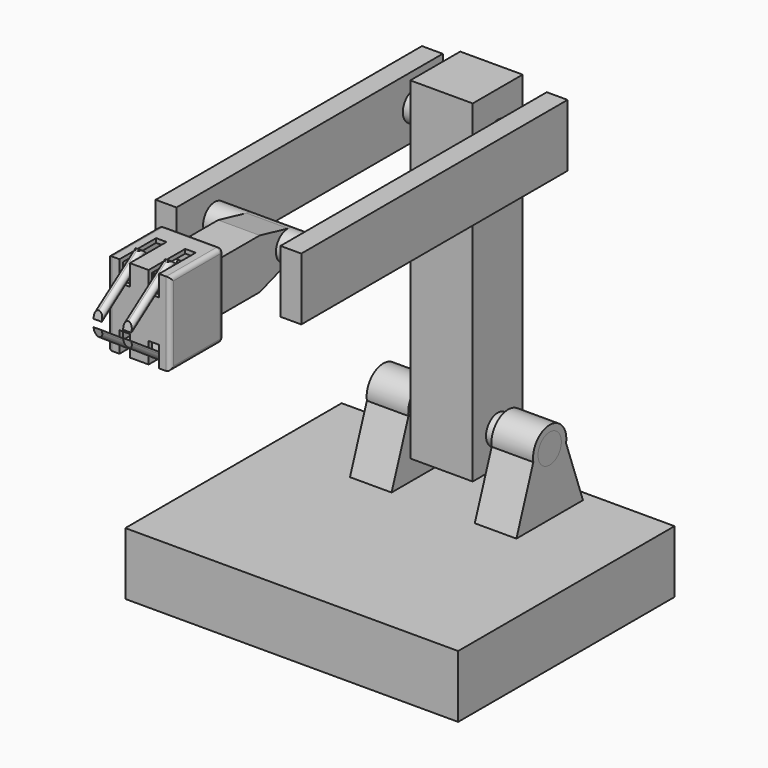
from build123d import *

# Parameters (mm, degrees)
F0_W      = 80
F0_H      = 65
F1_DEPTH  = 15
F3_R      = 3.5
F4_DEPTH  = 10
F6_R      = 3.5
F7_DEPTH  = 20
F8_W      = 15
F8_H      = 80
F9_DEPTH  = 7.5
F10_R     = 3.5
F11_DEPTH = 5
F12_R     = 3.5
F13_DEPTH = 5
F14_DEPTH = 10
F15_W     = 80
F15_H     = 15
F16_DEPTH = 5
F19_DEPTH = 5
F20_R     = 3.5
F21_DEPTH = 3
F22_R     = 3.5
F23_DEPTH = 3
F24_R     = 3.5
F25_DEPTH = 15.5
F26_R     = 3.25
F26_R_2   = 2.5
F27_DEPTH = 1
F28_DEPTH = 5
F30_W     = 15
F30_H     = 20
F31_DEPTH = 15
F32_R     = 2.5
F33_DEPTH = 7
F34_T     = -1
F35_R     = 3
F35_R_2   = 1.5
F36_DEPTH = 1
F37_R     = 3
F37_R_2   = 1.5
F38_DEPTH = 1
F39_R     = 3
F39_R_2   = 1.5
F40_DEPTH = 1
F41_R     = 3
F41_R_2   = 1.5
F42_DEPTH = 1
F44_DEPTH = 1.25
F45_DEPTH = 13
F47_DEPTH = 1.25
F48_DEPTH = 13
F49_W     = 2.5
F49_H     = 10
F50_DEPTH = 2
F51_DEPTH = 2
F53_R     = 1.5
F54_DEPTH = 1
F56_W     = 2.5
F56_H     = 10
F57_DEPTH = 2
F58_DEPTH = 2
F60_R     = 1.5
F61_DEPTH = 1
F64_DEPTH = 1
F65_R     = 0.99999
F65_2_R   = 0.99999
F65_3_R   = 0.99999
F65_4_R   = 0.99999
F65_5_R   = 0.99999


# Not quite as in the source:
# - a fillet or chamfer is up to 0.001 mm smaller than in the source, because OpenCascade refuses the exact size


with BuildPart() as f1:
    # F0 (on Top) → F1 (new body)
    with BuildSketch(Plane.XY):
        Rectangle(F0_W, F0_H)
    extrude(amount=F1_DEPTH)

    # F3 (on offset) → F4 (join)
    with BuildSketch(Plane.YZ.offset(10)):
        with BuildLine():
            ThreePointArc((24.9208571669, 29.113904778), (24.9801749886, 29.5551887112), (25, 30))
            ThreePointArc((25, 30), (19.5551887112, 34.9801749886), (15.0791428331, 29.113904778))
            ThreePointArc((15.0791428331, 29.113904778), (20, 25), (24.9208571669, 29.113904778))
        make_face()
        with Locations((20, 30)):
            Circle(F3_R, mode=Mode.SUBTRACT)
        with BuildLine():
            ThreePointArc((24.9208571669, 29.113904778), (20, 25), (15.0791428331, 29.113904778))
            Line((15.0791428331, 29.113904778), (10, 15))
            Line((10, 15), (30, 15))
            Line((30, 15), (24.9208571669, 29.113904778))
        make_face()
    extrude(amount=F4_DEPTH)

    # F5: F1 across plane


with BuildPart() as f1_1:
    add(f1.part)
    add(f1.part.mirror(Plane.YZ))


with BuildPart() as f7:
    # F6 (on Right) → F7 (new body, symmetric)
    with BuildSketch(Plane.YZ):
        with Locations((20, 30)):
            Circle(F6_R)
    extrude(amount=F7_DEPTH, both=True)

    # F8 (on Right) → F9 (join, symmetric)
    with BuildSketch(Plane.YZ):
        with Locations((20, 62)):
            Rectangle(F8_W, F8_H)
    extrude(amount=F9_DEPTH, both=True)

    # F10 (on face) → F11 (cut)
    with BuildSketch(Plane.YZ.offset(7.5)):
        with Locations((20, 92)):
            Circle(F10_R)
    extrude(amount=-F11_DEPTH, mode=Mode.SUBTRACT)

    # F12 (on face) → F13 (cut)
    with BuildSketch(Plane(origin=(-7.5, 0, 0), x_dir=(0, -1, 0), z_dir=(-1, 0, 0))):
        with Locations((-20, 92)):
            Circle(F12_R)
    extrude(amount=-F13_DEPTH, mode=Mode.SUBTRACT)


with BuildPart() as f14:
    # F14 (new): a face of the model
    f14_faces = [f7.part.faces().sort_by_distance(p)[0] for p in [
        (2.5, 20, 92),
    ]]
    extrude(f14_faces, amount=F14_DEPTH)

    # F15 (on face) → F16 (join)
    with BuildSketch(Plane.YZ.offset(12.5)):
        with Locations((-11.5, 92)):
            Rectangle(F15_W, F15_H)
    extrude(amount=F16_DEPTH)


with BuildPart() as f17_1:
    # F17: instance of F14
    add(f14.part.mirror(Plane.YZ))

    # F22 (on face) → F23 (cut)
    with BuildSketch(Plane.YZ.offset(-12.5)):
        with Locations((-40, 92.5)):
            Circle(F22_R)
    extrude(amount=-F23_DEPTH, mode=Mode.SUBTRACT)


with BuildPart() as f19:
    # F18 (on Right) → F19 (new body, symmetric)
    with BuildSketch(Plane.YZ):
        with BuildLine():
            ThreePointArc((-38.8863327684, 89.1819063761), (-37.1585360014, 90.4564534885), (-36.5, 92.5))
            ThreePointArc((-36.5, 92.5), (-37.0806183009, 94.4305984811), (-38.6298345687, 95.7206593565))
            Line((-38.6298345687, 95.7206593565), (-39.7982464523, 95.9941802338))
            ThreePointArc((-39.7982464523, 95.9941802338), (-43.4690563176, 92.0356205589), (-38.8863327684, 89.1819063761))
        make_face()
        with BuildLine():
            Line((-39.7982464523, 95.9941802338), (-38.6298345687, 95.7206593565))
            ThreePointArc((-38.6298345687, 95.7206593565), (-39.2022307748, 95.9078679938), (-39.7982464523, 95.9941802338))
        make_face()
        with BuildLine():
            Line((-48.3666002653, 86), (-38.8863327684, 89.1819063761))
            ThreePointArc((-38.8863327684, 89.1819063761), (-43.4690563176, 92.0356205589), (-39.7982464523, 95.9941802338))
            Line((-39.7982464523, 95.9941802338), (-48.3666002653, 98))
            Line((-48.3666002653, 98), (-60.3666002653, 98))
            Line((-60.3666002653, 98), (-60.3666002653, 86))
            Line((-60.3666002653, 86), (-48.3666002653, 86))
        make_face()
    extrude(amount=F19_DEPTH, both=True)

    # F24 (on Right) → F25 (join, symmetric)
    with BuildSketch(Plane.YZ):
        with Locations((-40, 92.5)):
            Circle(F24_R)
    extrude(amount=F25_DEPTH, both=True)

    # F26 (on face) → F27 (join)
    with BuildSketch(Plane.XZ.offset(60.3666002653)):
        with Locations((0, 92)):
            Circle(F26_R)
        with Locations((0, 92)):
            Circle(F26_R_2, mode=Mode.SUBTRACT)
    extrude(amount=F27_DEPTH)

    # F28 (cut): a face of the model
    f28_faces = [f19.faces().sort_by_distance(p)[0] for p in [
        (0, -60.3666002653, 92),
    ]]
    extrude(f28_faces, amount=-F28_DEPTH, mode=Mode.SUBTRACT)


with BuildPart() as f14_1:
    add(f14.part)

    # F20 (on face) → F21 (cut)
    with BuildSketch(Plane(origin=(12.5, 0, 0), x_dir=(0, -1, 0), z_dir=(-1, 0, 0))):
        with Locations((40, 92.5)):
            Circle(F20_R)
    extrude(amount=-F21_DEPTH, mode=Mode.SUBTRACT)


with BuildPart() as f31:
    # F30 (on offset) → F31 (new body)
    with BuildSketch(Plane.XZ.offset(62.3666002653)):
        with Locations((0, 92)):
            Rectangle(F30_W, F30_H)
    extrude(amount=F31_DEPTH)

    # F32 (on face) → F33 (join, through all)
    with BuildSketch(Plane(origin=(0, -62.3666002653, 0), x_dir=(-1, 0, 0), z_dir=(0, 1, 0))):
        with Locations((0, 92)):
            Circle(F32_R)
    extrude(amount=F33_DEPTH)

    # F34
    f34_openings = [f31.faces().sort_by_distance(p)[0] for p in [
        (0, -77.3666, 92),
    ]]
    offset(amount=F34_T, openings=f34_openings, kind=Kind.INTERSECTION)

    # F35 (on face) → F36 (join)
    with BuildSketch(Plane.YZ.offset(-6.5)):
        with Locations((-70.3666002653, 96)):
            Circle(F35_R)
        with Locations((-70.3666002653, 96)):
            Circle(F35_R_2, mode=Mode.SUBTRACT)
    extrude(amount=F36_DEPTH)

    # F37 (on face) → F38 (join)
    with BuildSketch(Plane(origin=(6.5, 0, 0), x_dir=(0, -1, 0), z_dir=(-1, 0, 0))):
        with Locations((70.3666002653, 96)):
            Circle(F37_R)
        with Locations((70.3666002653, 96)):
            Circle(F37_R_2, mode=Mode.SUBTRACT)
    extrude(amount=F38_DEPTH)

    # F39 (on face) → F40 (join)
    with BuildSketch(Plane.YZ.offset(-6.5)):
        with Locations((-70.3666002653, 88)):
            Circle(F39_R)
        with Locations((-70.3666002653, 88)):
            Circle(F39_R_2, mode=Mode.SUBTRACT)
    extrude(amount=F40_DEPTH)

    # F41 (on face) → F42 (join)
    with BuildSketch(Plane(origin=(6.5, 0, 0), x_dir=(0, -1, 0), z_dir=(-1, 0, 0))):
        with Locations((70.3666002653, 88)):
            Circle(F41_R)
        with Locations((70.3666002653, 88)):
            Circle(F41_R_2, mode=Mode.SUBTRACT)
    extrude(amount=F42_DEPTH)


with BuildPart() as f44:
    # F43 (on Right) → F44 (new body, symmetric)
    with BuildSketch(Plane.YZ):
        with BuildLine():
            ThreePointArc((-67.3727136422, 95.8085766788), (-67.3681289991, 95.904239542), (-67.3666002653, 96))
            ThreePointArc((-67.3666002653, 96), (-67.3681289991, 96.095760458), (-67.3727136422, 96.1914233212))
            ThreePointArc((-67.3727136422, 96.1914233212), (-67.5134307165, 96.9270509831), (-67.8319793028, 97.6048976841))
            ThreePointArc((-67.8319793028, 97.6048976841), (-67.9395492822, 97.7633557569), (-68.0570109132, 97.9146271241))
            ThreePointArc((-68.0570109132, 97.9146271241), (-68.6032445085, 98.4270509831), (-69.2593840225, 98.7882023226))
            ThreePointArc((-69.2593840225, 98.7882023226), (-69.4395492822, 98.8531695489), (-69.6234928166, 98.9065084413))
            ThreePointArc((-69.6234928166, 98.9065084413), (-70.3666002653, 99), (-71.1097077141, 98.9065084413))
            ThreePointArc((-71.1097077141, 98.9065084413), (-71.2936512485, 98.8531695489), (-71.4738165082, 98.7882023226))
            ThreePointArc((-71.4738165082, 98.7882023226), (-72.1299560222, 98.4270509831), (-72.6761896175, 97.9146271241))
            ThreePointArc((-72.6761896175, 97.9146271241), (-72.7936512485, 97.7633557569), (-72.9012212278, 97.6048976841))
            ThreePointArc((-72.9012212278, 97.6048976841), (-73.2197698142, 96.9270509831), (-73.3604868885, 96.1914233212))
            ThreePointArc((-73.3604868885, 96.1914233212), (-73.3666002653, 96), (-73.3604868885, 95.8085766788))
            ThreePointArc((-73.3604868885, 95.8085766788), (-73.2197698142, 95.0729490169), (-72.9012212278, 94.3951023159))
            ThreePointArc((-72.9012212278, 94.3951023159), (-72.7936512485, 94.2366442431), (-72.6761896175, 94.0853728759))
            ThreePointArc((-72.6761896175, 94.0853728759), (-72.1299560222, 93.5729490169), (-71.4738165082, 93.2117976774))
            ThreePointArc((-71.4738165082, 93.2117976774), (-71.2936512485, 93.1468304511), (-71.1097077141, 93.0934915587))
            ThreePointArc((-71.1097077141, 93.0934915587), (-70.3666002653, 93), (-69.6234928166, 93.0934915587))
            ThreePointArc((-69.6234928166, 93.0934915587), (-69.4395492822, 93.1468304511), (-69.2593840225, 93.2117976774))
            ThreePointArc((-69.2593840225, 93.2117976774), (-68.6032445085, 93.5729490169), (-68.0570109132, 94.0853728759))
            ThreePointArc((-68.0570109132, 94.0853728759), (-67.9395492822, 94.2366442431), (-67.8319793028, 94.3951023159))
            ThreePointArc((-67.8319793028, 94.3951023159), (-67.5134307165, 95.0729490169), (-67.3727136422, 95.8085766788))
        make_face()
        with BuildLine():
            ThreePointArc((-67.8319793028, 97.6048976841), (-67.5134307165, 96.9270509831), (-67.3727136422, 96.1914233212))
            Line((-67.3727136422, 96.1914233212), (-66.1365870122, 96.8486835091))
            Line((-66.1365870122, 96.8486835091), (-66.2910955094, 97.3242117673))
            Line((-66.2910955094, 97.3242117673), (-66.4456040066, 97.7997400254))
            Line((-66.4456040066, 97.7997400254), (-67.8319793028, 97.6048976841))
        make_face()
        with BuildLine():
            Line((-66.1365870122, 95.1513164909), (-67.3727136422, 95.8085766788))
            ThreePointArc((-67.3727136422, 95.8085766788), (-67.5134307165, 95.0729490169), (-67.8319793028, 94.3951023159))
            Line((-67.8319793028, 94.3951023159), (-66.4456040066, 94.2002599746))
            Line((-66.4456040066, 94.2002599746), (-66.2910955094, 94.6757882327))
            Line((-66.2910955094, 94.6757882327), (-66.1365870122, 95.1513164909))
        make_face()
        with BuildLine():
            ThreePointArc((-69.2593840225, 98.7882023226), (-68.6032445085, 98.4270509831), (-68.0570109132, 97.9146271241))
            Line((-68.0570109132, 97.9146271241), (-67.4432913077, 99.1729387889))
            Line((-67.4432913077, 99.1729387889), (-67.8477998049, 99.4668314151))
            Line((-67.8477998049, 99.4668314151), (-68.252308302, 99.7607240412))
            Line((-68.252308302, 99.7607240412), (-69.2593840225, 98.7882023226))
        make_face()
        with BuildLine():
            Line((-67.4432913077, 92.8270612111), (-68.0570109132, 94.0853728759))
            ThreePointArc((-68.0570109132, 94.0853728759), (-68.6032445085, 93.5729490169), (-69.2593840225, 93.2117976774))
            Line((-69.2593840225, 93.2117976774), (-68.252308302, 92.2392759588))
            Line((-68.252308302, 92.2392759588), (-67.8477998049, 92.5331685849))
            Line((-67.8477998049, 92.5331685849), (-67.4432913077, 92.8270612111))
        make_face()
        with BuildLine():
            ThreePointArc((-71.1097077141, 98.9065084413), (-70.3666002653, 99), (-69.6234928166, 98.9065084413))
            Line((-69.6234928166, 98.9065084413), (-69.8666002653, 100.2852392956))
            Line((-69.8666002653, 100.2852392956), (-70.3666002653, 100.2852392956))
            Line((-70.3666002653, 100.2852392956), (-70.8666002653, 100.2852392956))
            Line((-70.8666002653, 100.2852392956), (-71.1097077141, 98.9065084413))
        make_face()
        with BuildLine():
            Line((-69.8666002653, 91.7147607044), (-69.6234928166, 93.0934915587))
            ThreePointArc((-69.6234928166, 93.0934915587), (-70.3666002653, 93), (-71.1097077141, 93.0934915587))
            Line((-71.1097077141, 93.0934915587), (-70.8666002653, 91.7147607044))
            Line((-70.8666002653, 91.7147607044), (-70.3666002653, 91.7147607044))
            Line((-70.3666002653, 91.7147607044), (-69.8666002653, 91.7147607044))
        make_face()
        with BuildLine():
            ThreePointArc((-72.6761896175, 97.9146271241), (-72.1299560222, 98.4270509831), (-71.4738165082, 98.7882023226))
            Line((-71.4738165082, 98.7882023226), (-72.4808922286, 99.7607240412))
            Line((-72.4808922286, 99.7607240412), (-72.8854007258, 99.4668314151))
            Line((-72.8854007258, 99.4668314151), (-73.289909223, 99.1729387889))
            Line((-73.289909223, 99.1729387889), (-72.6761896175, 97.9146271241))
        make_face()
        with BuildLine():
            Line((-72.4808922286, 92.2392759588), (-71.4738165082, 93.2117976774))
            ThreePointArc((-71.4738165082, 93.2117976774), (-72.1299560222, 93.5729490169), (-72.6761896175, 94.0853728759))
            Line((-72.6761896175, 94.0853728759), (-73.289909223, 92.8270612111))
            Line((-73.289909223, 92.8270612111), (-72.8854007258, 92.5331685849))
            Line((-72.8854007258, 92.5331685849), (-72.4808922286, 92.2392759588))
        make_face()
        with BuildLine():
            ThreePointArc((-73.3604868885, 96.1914233212), (-73.2197698142, 96.9270509831), (-72.9012212278, 97.6048976841))
            Line((-72.9012212278, 97.6048976841), (-74.2875965241, 97.7997400254))
            Line((-74.2875965241, 97.7997400254), (-74.4421050213, 97.3242117673))
            Line((-74.4421050213, 97.3242117673), (-74.5966135185, 96.8486835091))
            Line((-74.5966135185, 96.8486835091), (-73.3604868885, 96.1914233212))
        make_face()
        with BuildLine():
            Line((-74.2875965241, 94.2002599746), (-72.9012212278, 94.3951023159))
            ThreePointArc((-72.9012212278, 94.3951023159), (-73.2197698142, 95.0729490169), (-73.3604868885, 95.8085766788))
            Line((-73.3604868885, 95.8085766788), (-74.5966135185, 95.1513164909))
            Line((-74.5966135185, 95.1513164909), (-74.4421050213, 94.6757882327))
            Line((-74.4421050213, 94.6757882327), (-74.2875965241, 94.2002599746))
        make_face()
    extrude(amount=F44_DEPTH, both=True)

    # F45 (add): a face of the model
    f45_faces = [f31.part.faces().sort_by_distance(p)[0] for p in [
        (6.5, -70.3666002653, 96),
    ]]
    extrude(f45_faces, amount=F45_DEPTH)


with BuildPart() as f47:
    # F46 (on Right) → F47 (new body, symmetric)
    with BuildSketch(Plane.YZ):
        with BuildLine():
            ThreePointArc((-67.460091824, 87.2568925513), (-67.39006492, 87.6255172394), (-67.3666002653, 88))
            ThreePointArc((-67.3666002653, 88), (-67.39006492, 88.3744827606), (-67.460091824, 88.7431074487))
            ThreePointArc((-67.460091824, 88.7431074487), (-67.5134307165, 88.9270509831), (-67.5783979428, 89.1072162428))
            ThreePointArc((-67.5783979428, 89.1072162428), (-67.9395492822, 89.7633557569), (-68.4519731412, 90.3095893522))
            ThreePointArc((-68.4519731412, 90.3095893522), (-68.6032445085, 90.4270509831), (-68.7617025812, 90.5346209625))
            ThreePointArc((-68.7617025812, 90.5346209625), (-69.4395492822, 90.8531695489), (-70.1751769441, 90.9938866231))
            ThreePointArc((-70.1751769441, 90.9938866231), (-70.3666002653, 91), (-70.5580235866, 90.9938866231))
            ThreePointArc((-70.5580235866, 90.9938866231), (-71.2936512485, 90.8531695489), (-71.9714979494, 90.5346209625))
            ThreePointArc((-71.9714979494, 90.5346209625), (-72.1299560222, 90.4270509831), (-72.2812273895, 90.3095893522))
            ThreePointArc((-72.2812273895, 90.3095893522), (-72.7936512485, 89.7633557569), (-73.1548025879, 89.1072162428))
            ThreePointArc((-73.1548025879, 89.1072162428), (-73.2197698142, 88.9270509831), (-73.2731087067, 88.7431074487))
            ThreePointArc((-73.2731087067, 88.7431074487), (-73.3666002653, 88), (-73.2731087067, 87.2568925513))
            ThreePointArc((-73.2731087067, 87.2568925513), (-73.2197698142, 87.0729490169), (-73.1548025879, 86.8927837572))
            ThreePointArc((-73.1548025879, 86.8927837572), (-72.7936512485, 86.2366442431), (-72.2812273895, 85.6904106478))
            ThreePointArc((-72.2812273895, 85.6904106478), (-72.1299560222, 85.5729490169), (-71.9714979494, 85.4653790375))
            ThreePointArc((-71.9714979494, 85.4653790375), (-71.2936512485, 85.1468304511), (-70.5580235866, 85.0061133769))
            ThreePointArc((-70.5580235866, 85.0061133769), (-70.3666002653, 85), (-70.1751769441, 85.0061133769))
            ThreePointArc((-70.1751769441, 85.0061133769), (-69.4395492822, 85.1468304511), (-68.7617025812, 85.4653790375))
            ThreePointArc((-68.7617025812, 85.4653790375), (-68.6032445085, 85.5729490169), (-68.4519731412, 85.6904106478))
            ThreePointArc((-68.4519731412, 85.6904106478), (-67.9395492822, 86.2366442431), (-67.5783979428, 86.8927837572))
            ThreePointArc((-67.5783979428, 86.8927837572), (-67.5134307165, 87.0729490169), (-67.460091824, 87.2568925513))
        make_face()
        with BuildLine():
            ThreePointArc((-67.460091824, 88.7431074487), (-67.39006492, 88.3744827606), (-67.3666002653, 88))
            ThreePointArc((-67.3666002653, 88), (-67.39006492, 87.6255172394), (-67.460091824, 87.2568925513))
            Line((-67.460091824, 87.2568925513), (-66.0813609698, 87.5))
            Line((-66.0813609698, 87.5), (-66.0813609698, 88))
            Line((-66.0813609698, 88), (-66.0813609698, 88.5))
            Line((-66.0813609698, 88.5), (-67.460091824, 88.7431074487))
        make_face()
        with BuildLine():
            ThreePointArc((-68.4519731412, 90.3095893522), (-67.9395492822, 89.7633557569), (-67.5783979428, 89.1072162428))
            Line((-67.5783979428, 89.1072162428), (-66.6058762241, 90.1142919633))
            Line((-66.6058762241, 90.1142919633), (-66.8997688503, 90.5188004605))
            Line((-66.8997688503, 90.5188004605), (-67.1936614764, 90.9233089577))
            Line((-67.1936614764, 90.9233089577), (-68.4519731412, 90.3095893522))
        make_face()
        with BuildLine():
            Line((-66.6058762241, 85.8857080367), (-67.5783979428, 86.8927837572))
            ThreePointArc((-67.5783979428, 86.8927837572), (-67.9395492822, 86.2366442431), (-68.4519731412, 85.6904106478))
            Line((-68.4519731412, 85.6904106478), (-67.1936614764, 85.0766910423))
            Line((-67.1936614764, 85.0766910423), (-66.8997688503, 85.4811995395))
            Line((-66.8997688503, 85.4811995395), (-66.6058762241, 85.8857080367))
        make_face()
        with BuildLine():
            ThreePointArc((-70.1751769441, 90.9938866231), (-69.4395492822, 90.8531695489), (-68.7617025812, 90.5346209625))
            Line((-68.7617025812, 90.5346209625), (-68.5668602399, 91.9209962587))
            Line((-68.5668602399, 91.9209962587), (-69.042388498, 92.0755047559))
            Line((-69.042388498, 92.0755047559), (-69.5179167562, 92.2300132531))
            Line((-69.5179167562, 92.2300132531), (-70.1751769441, 90.9938866231))
        make_face()
        with BuildLine():
            Line((-68.5668602399, 84.0790037413), (-68.7617025812, 85.4653790375))
            ThreePointArc((-68.7617025812, 85.4653790375), (-69.4395492822, 85.1468304511), (-70.1751769441, 85.0061133769))
            Line((-70.1751769441, 85.0061133769), (-69.5179167562, 83.7699867469))
            Line((-69.5179167562, 83.7699867469), (-69.042388498, 83.9244952441))
            Line((-69.042388498, 83.9244952441), (-68.5668602399, 84.0790037413))
        make_face()
        with BuildLine():
            ThreePointArc((-71.9714979494, 90.5346209625), (-71.2936512485, 90.8531695489), (-70.5580235866, 90.9938866231))
            Line((-70.5580235866, 90.9938866231), (-71.2152837745, 92.2300132531))
            Line((-71.2152837745, 92.2300132531), (-71.6908120326, 92.0755047559))
            Line((-71.6908120326, 92.0755047559), (-72.1663402908, 91.9209962587))
            Line((-72.1663402908, 91.9209962587), (-71.9714979494, 90.5346209625))
        make_face()
        with BuildLine():
            Line((-71.2152837745, 83.7699867469), (-70.5580235866, 85.0061133769))
            ThreePointArc((-70.5580235866, 85.0061133769), (-71.2936512485, 85.1468304511), (-71.9714979494, 85.4653790375))
            Line((-71.9714979494, 85.4653790375), (-72.1663402908, 84.0790037413))
            Line((-72.1663402908, 84.0790037413), (-71.6908120326, 83.9244952441))
            Line((-71.6908120326, 83.9244952441), (-71.2152837745, 83.7699867469))
        make_face()
        with BuildLine():
            ThreePointArc((-73.1548025879, 89.1072162428), (-72.7936512485, 89.7633557569), (-72.2812273895, 90.3095893522))
            Line((-72.2812273895, 90.3095893522), (-73.5395390543, 90.9233089577))
            Line((-73.5395390543, 90.9233089577), (-73.8334316804, 90.5188004605))
            Line((-73.8334316804, 90.5188004605), (-74.1273243066, 90.1142919633))
            Line((-74.1273243066, 90.1142919633), (-73.1548025879, 89.1072162428))
        make_face()
        with BuildLine():
            Line((-73.5395390543, 85.0766910423), (-72.2812273895, 85.6904106478))
            ThreePointArc((-72.2812273895, 85.6904106478), (-72.7936512485, 86.2366442431), (-73.1548025879, 86.8927837572))
            Line((-73.1548025879, 86.8927837572), (-74.1273243066, 85.8857080367))
            Line((-74.1273243066, 85.8857080367), (-73.8334316804, 85.4811995395))
            Line((-73.8334316804, 85.4811995395), (-73.5395390543, 85.0766910423))
        make_face()
        with BuildLine():
            ThreePointArc((-73.2731087067, 87.2568925513), (-73.3666002653, 88), (-73.2731087067, 88.7431074487))
            Line((-73.2731087067, 88.7431074487), (-74.6518395609, 88.5))
            Line((-74.6518395609, 88.5), (-74.6518395609, 88))
            Line((-74.6518395609, 88), (-74.6518395609, 87.5))
            Line((-74.6518395609, 87.5), (-73.2731087067, 87.2568925513))
        make_face()
    extrude(amount=F47_DEPTH, both=True)

    # F39 (on face) → F48 (join)
    with BuildSketch(Plane.YZ.offset(-6.5)):
        with Locations((-70.3666002653, 88)):
            Circle(F39_R_2)
    extrude(amount=F48_DEPTH)


with BuildPart() as f31_1:
    add(f31.part)

    # F49 (on face) → F50 (cut)
    with BuildSketch(Plane.XY.offset(102)):
        with Locations((-3.45, -72.3666002653)):
            Rectangle(F49_W, F49_H)
    extrude(amount=-F50_DEPTH, mode=Mode.SUBTRACT)

    # F49 (on face) → F51 (cut)
    with BuildSketch(Plane.XY.offset(102)):
        with Locations((3.55, -72.3666002653)):
            Rectangle(F49_W, F49_H)
    extrude(amount=-F51_DEPTH, mode=Mode.SUBTRACT)

    # F56 (on face) → F57 (cut)
    with BuildSketch(Plane(origin=(0, 0, 82), x_dir=(1, 0, 0), z_dir=(0, 0, -1))):
        with Locations((-3.45, 72.3666002653)):
            Rectangle(F56_W, F56_H)
    extrude(amount=-F57_DEPTH, mode=Mode.SUBTRACT)

    # F56 (on face) → F58 (cut)
    with BuildSketch(Plane(origin=(0, 0, 82), x_dir=(1, 0, 0), z_dir=(0, 0, -1))):
        with Locations((3.55, 72.3666002653)):
            Rectangle(F56_W, F56_H)
    extrude(amount=-F58_DEPTH, mode=Mode.SUBTRACT)

    # F63 (on face) → F64 (join)
    with BuildSketch(Plane.XZ.offset(77.3666002653)):
        Polygon((-4.7, 102), (-7.5, 102), (-7.5, 82), (-4.7, 82), (-4.7, 87), (-2.2, 87), (-2.2, 82), (2.3, 82), (2.3, 87), (4.8, 87), (4.8, 82), (7.5, 82), (7.5, 102), (4.8, 102), (4.8, 97), (2.3, 97), (2.3, 102), (-2.2, 102), (-2.2, 97), (-4.7, 97), align=None)
    extrude(amount=F64_DEPTH)

    # F65 (radius 1 in the source; OpenCascade refuses exactly that, so slightly less here)
    f65_edges = [f31_1.edges().sort_by_distance(p)[0] for p in [
        (7.5, -70.3666, 102),
        (7.5, -70.3666, 82),
        (-7.5, -70.3666, 102),
        (-7.5, -70.3666, 82),
        (7.5, -78.3666, 92),
        (-7.5, -78.3666, 92),
        (0, -62.3666, 102),
        (0, -62.3666, 82),
        (7.5, -62.3666, 92),
        (-7.5, -62.3666, 92),
    ]]
    fillet(f65_edges, radius=F65_R)


with BuildPart() as f54:
    # F53 (on offset) → F54 (new body, symmetric)
    with BuildSketch(Plane.YZ.offset(3.55)):
        with BuildLine():
            ThreePointArc((-72.4732790486, 98.1358615368), (-71.5241761052, 93.232326216), (-67.3666002653, 96))
            ThreePointArc((-67.3666002653, 96), (-68.2607906925, 98.1367185221), (-70.4103109606, 98.9996815456))
            ThreePointArc((-70.4103109606, 98.9996815456), (-71.5253021162, 98.7672025623), (-72.4732790486, 98.1358615368))
        make_face()
        with Locations((-70.3666002653, 96)):
            Circle(F53_R, mode=Mode.SUBTRACT)
        with BuildLine():
            ThreePointArc((-72.4732790486, 98.1358615368), (-71.5253021162, 98.7672025623), (-70.4103109606, 98.9996815456))
            Line((-70.4103109606, 98.9996815456), (-74.1552655241, 103.0277474981))
            Line((-74.1552655241, 103.0277474981), (-86.0059894049, 94.6724890639))
            Line((-86.0059894049, 94.6724890639), (-86.3666002653, 92.7052677222))
            Line((-86.3666002653, 92.7052677222), (-74.9245220356, 100.7724137965))
            Line((-74.9245220356, 100.7724137965), (-72.4732790486, 98.1358615368))
        make_face()
    extrude(amount=F54_DEPTH, both=True)


with BuildPart() as f55_1:
    # F55: instance of F54
    add(f54.part.mirror(Plane.YZ))

    # F65#3 (radius 1 in the source; OpenCascade refuses exactly that, so slightly less here)
    f65_3_edges = [f55_1.edges().sort_by_distance(p)[0] for p in [
        (-4.55, -80.080627, 98.850118),
        (-2.55, -80.080627, 98.850118),
        (-3.55, -74.155266, 103.027747),
    ]]
    fillet(f65_3_edges, radius=F65_3_R)


with BuildPart() as f61:
    # F60 (on offset) → F61 (new body, symmetric)
    with BuildSketch(Plane.YZ.offset(3.55)):
        with BuildLine():
            ThreePointArc((-70.3666002653, 85), (-68.2452799218, 85.8786796564), (-67.3666002653, 88))
            ThreePointArc((-67.3666002653, 88), (-71.5523418734, 90.7557243765), (-72.429278158, 85.8216152977))
            ThreePointArc((-72.429278158, 85.8216152977), (-71.4767457272, 85.2129626746), (-70.3666002653, 85))
        make_face()
        with Locations((-70.3666002653, 88)):
            Circle(F60_R, mode=Mode.SUBTRACT)
        with BuildLine():
            ThreePointArc((-70.3666002653, 85), (-71.4767457272, 85.2129626746), (-72.429278158, 85.8216152977))
            Line((-72.429278158, 85.8216152977), (-74.7751712589, 83.0909037496))
            Line((-74.7751712589, 83.0909037496), (-86.3666002653, 90.9419402155))
            Line((-86.3666002653, 90.9419402155), (-85.9361075752, 88.9888206484))
            Line((-85.9361075752, 88.9888206484), (-73.950603614, 80.8280795793))
            Line((-73.950603614, 80.8280795793), (-70.3666002653, 85))
        make_face()
    extrude(amount=F61_DEPTH, both=True)


with BuildPart() as f62_1:
    # F62: instance of F61
    add(f61.part.mirror(Plane.YZ))

    # F65#5 (radius 1 in the source; OpenCascade refuses exactly that, so slightly less here)
    f65_5_edges = [f62_1.edges().sort_by_distance(p)[0] for p in [
        (-2.55, -79.943356, 84.90845),
        (-4.55, -79.943356, 84.90845),
        (-3.55, -73.950604, 80.82808),
    ]]
    fillet(f65_5_edges, radius=F65_5_R)


with BuildPart() as f54_1:
    add(f54.part)

    # F65#2 (radius 1 in the source; OpenCascade refuses exactly that, so slightly less here)
    f65_2_edges = [f54_1.edges().sort_by_distance(p)[0] for p in [
        (3.55, -74.155266, 103.027747),
        (4.55, -80.080627, 98.850118),
        (2.55, -80.080627, 98.850118),
    ]]
    fillet(f65_2_edges, radius=F65_2_R)


with BuildPart() as f61_1:
    add(f61.part)

    # F65#4 (radius 1 in the source; OpenCascade refuses exactly that, so slightly less here)
    f65_4_edges = [f61_1.edges().sort_by_distance(p)[0] for p in [
        (4.55, -79.943356, 84.90845),
        (2.55, -79.943356, 84.90845),
        (3.55, -73.950604, 80.82808),
        (3.55, -85.936108, 88.988821),
    ]]
    fillet(f65_4_edges, radius=F65_4_R)


solid = Compound([f1_1.part, f7.part, f17_1.part, f19.part, f14_1.part, f44.part, f47.part, f31_1.part, f55_1.part, f62_1.part, f54_1.part, f61_1.part])
